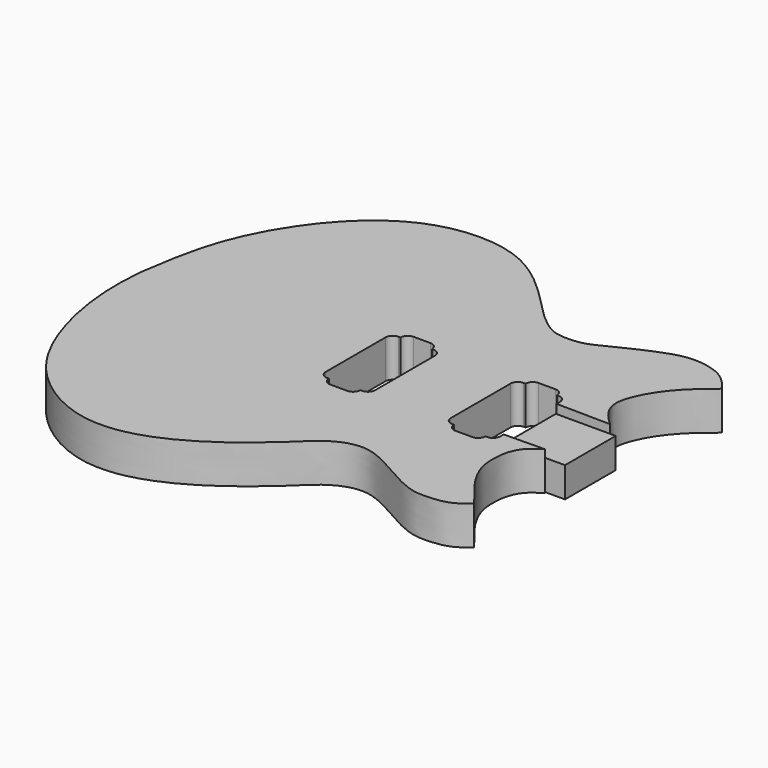
from build123d import *

# Parameters (mm, degrees)
F1_DEPTH = 32
F2_DEPTH = 25


# Not quite as in the source:
# - the dataset's text gives a spline's control points without its knots; the knots are read off the source's solid


with BuildPart() as f1:
    # F0 (on Top) → F1 (new body)
    with BuildSketch(Plane.XY):
        with BuildLine():
            Line((128.11855, -26.992556), (128.11855, -30.537747))
            ThreePointArc((128.11855, -30.537747), (126.3611906871, -34.7803876871), (122.11855, -36.537747))
            Line((122.11855, -36.537747), (120.61855, -36.537747))
            ThreePointArc((120.61855, -36.537747), (118.8611906871, -40.7803876871), (114.61855, -42.537747))
            Line((114.61855, -42.537747), (100.61855, -42.537747))
            ThreePointArc((100.61855, -42.537747), (96.3759093129, -40.7803876871), (94.61855, -36.537747))
            Line((94.61855, -36.537747), (93.11855, -36.537747))
            ThreePointArc((93.11855, -36.537747), (88.8759093129, -34.7803876871), (87.11855, -30.537747))
            Line((87.11855, -30.537747), (87.11855, -27.571379))
            Line((87.11855, -27.571379), (87.11855, 28.420645))
            Line((87.11855, 28.420645), (87.11855, 31.375222))
            ThreePointArc((87.11855, 31.375222), (88.8759093129, 35.6178626871), (93.11855, 37.375222))
            Line((93.11855, 37.375222), (94.795262, 37.375222))
            ThreePointArc((94.795262, 37.375222), (96.5526213129, 41.6178626871), (100.795262, 43.375222))
            Line((100.795262, 43.375222), (114.795262, 43.375222))
            ThreePointArc((114.795262, 43.375222), (119.0379026871, 41.6178626871), (120.795262, 37.375222))
            Line((120.795262, 37.375222), (122.11855, 37.375222))
            ThreePointArc((122.11855, 37.375222), (126.3611906871, 35.6178626871), (128.11855, 31.375222))
            Line((128.11855, 31.375222), (128.11855, 27.841822))
            Line((128.11855, 27.841822), (172.9125551406, 27.2094361451))
            Line((172.9125551406, 27.2094361451), (172.66942, 27.424633))
            add(Edge.make_bspline(
                [(172.66942, 27.424633), (167.871034, 31.997809), (160.884208, 38.656711), (156.137415, 53.284463), (160.193035, 66.023078), (167.169802, 79.755438), (176.387559, 91.559743), (185.682788, 100.843754), (193.506128, 106.220487), (196.785168, 109.649245), (198.273954, 111.206008)],
                knots=[0, 0, 0, 0, 19.531082, 28.438782, 44.550618, 57.575462, 74.948895, 89.097271, 96.849551, 103.296396, 103.296396, 103.296396, 103.296396], degree=3))
            add(Edge.make_bspline(
                [(198.273954, 111.206008), (196.74345, 113.286069), (192.72903, 118.741945), (184.267476, 126.325497), (171.232678, 130.863282), (156.327424, 132.557046), (141.22601, 128.653616), (129.589308, 123.81371), (122.98281, 120.84288), (120.850652, 119.884084)],
                knots=[0, 0, 0, 0, 7.752281, 20.333776, 33.316696, 48.528894, 64.672537, 79.38681, 86.398606, 86.398606, 86.398606, 86.398606], degree=3))
            add(Edge.make_bspline(
                [(-197.316872, 3.566186), (-194.151047, 24.719101), (-188.108701, 65.091897), (-162.021967, 116.352781), (-130.86328, 152.302836), (-96.724552, 173.761687), (-59.74996, 181.547686), (-22.564565, 176.180637), (9.419666, 155.063229), (33.501098, 130.558185), (51.25784, 112.141003), (66.286047, 104.0853), (76.605316, 103.319713), (90.886431, 104.777025), (104.655638, 112.220648), (115.413772, 117.311368), (120.850652, 119.884084)],
                knots=[0, 0, 0, 0, 63.802519, 121.774521, 169.773876, 205.019419, 240.682587, 281.141136, 313.95816, 353.572334, 384.673433, 389.550292, 404.393012, 414.645616, 432.369939, 450.479395, 450.479395, 450.479395, 450.479395], degree=3))
            add(Edge.make_bspline(
                [(-197.316872, 3.566186), (-197.624379, -0.637733), (-198.295725, -9.815665), (-198.647796, -34.467428), (-194.485064, -67.579456), (-182.691117, -104.966855), (-164.677096, -138.124332), (-136.165814, -164.979956), (-102.762876, -179.368608), (-71.00728, -179.454967), (-37.05201, -169.30943), (-2.493851, -147.271936), (24.466834, -123.742322), (41.285505, -107.204016), (54.138554, -99.786791), (72.056904, -96.350074), (93.649355, -105.943556), (113.748436, -118.640374), (132.940688, -126.602188), (147.568962, -126.099418), (159.302165, -124.576547), (167.708274, -119.626164), (171.919796, -116.165392), (173.668353, -114.728534)],
                knots=[0, 0, 0, 0, 12.643441, 27.602973, 73.919947, 111.968744, 144.719609, 186.038741, 227.285303, 250.224144, 279.988368, 332.317829, 371.677854, 387.410033, 402.892165, 415.53479, 440.623239, 470.206225, 488.287081, 501.329992, 513.703212, 523.278344, 530.076107, 530.076107, 530.076107, 530.076107], degree=3))
            add(Edge.make_bspline(
                [(161.7935, -26.575367), (158.372259, -28.734199), (151.617288, -32.996644), (145.431621, -43.870551), (144.017132, -55.890765), (144.524139, -69.926976), (150.737184, -84.166536), (159.643929, -97.29374), (168.095078, -106.690173), (172.207415, -112.621416), (173.668353, -114.728534)],
                knots=[0, 0, 0, 0, 11.991106, 23.675499, 35.981856, 47.965187, 65.410279, 81.577072, 95.529288, 103.217047, 103.217047, 103.217047, 103.217047], degree=3))
            Line((161.7935, -26.575367), (161.8852475749, -26.5158497567))
            Line((161.8852475749, -26.5158497567), (128.11855, -26.992556))
        make_face()
        with BuildLine():
            ThreePointArc((-8.806872, 37.375222), (-7.0495126871, 41.6178626871), (-2.806872, 43.375222))
            Line((-2.806872, 43.375222), (11.193128, 43.375222))
            ThreePointArc((11.193128, 43.375222), (15.4357686871, 41.6178626871), (17.193128, 37.375222))
            Line((17.193128, 37.375222), (18.516416, 37.375222))
            ThreePointArc((18.516416, 37.375222), (22.7590566871, 35.6178626871), (24.516416, 31.375222))
            Line((24.516416, 31.375222), (24.516416, -30.537747))
            ThreePointArc((24.516416, -30.537747), (22.7590566871, -34.7803876871), (18.516416, -36.537747))
            Line((18.516416, -36.537747), (17.016416, -36.537747))
            ThreePointArc((17.016416, -36.537747), (15.2590566871, -40.7803876871), (11.016416, -42.537747))
            Line((11.016416, -42.537747), (-2.983584, -42.537747))
            ThreePointArc((-2.983584, -42.537747), (-7.2262246871, -40.7803876871), (-8.983584, -36.537747))
            Line((-8.983584, -36.537747), (-10.483584, -36.537747))
            ThreePointArc((-10.483584, -36.537747), (-14.7262246871, -34.7803876871), (-16.483584, -30.537747))
            Line((-16.483584, -30.537747), (-16.483584, 31.375222))
            ThreePointArc((-16.483584, 31.375222), (-14.7262246871, 35.6178626871), (-10.483584, 37.375222))
            Line((-10.483584, 37.375222), (-8.806872, 37.375222))
        make_face(mode=Mode.SUBTRACT)
    extrude(amount=F1_DEPTH)


with BuildPart() as f2:
    # F0 (on Top) → F2 (new body)
    with BuildSketch(Plane.XY):
        Polygon((128.11855, -17.581263), (128.11855, -25.354135), (177.649687, -25.354135), (177.649687, 27.142559), (128.11855, 27.142559), align=None)
    extrude(amount=F2_DEPTH)


solid = Compound([f1.part, f2.part])
